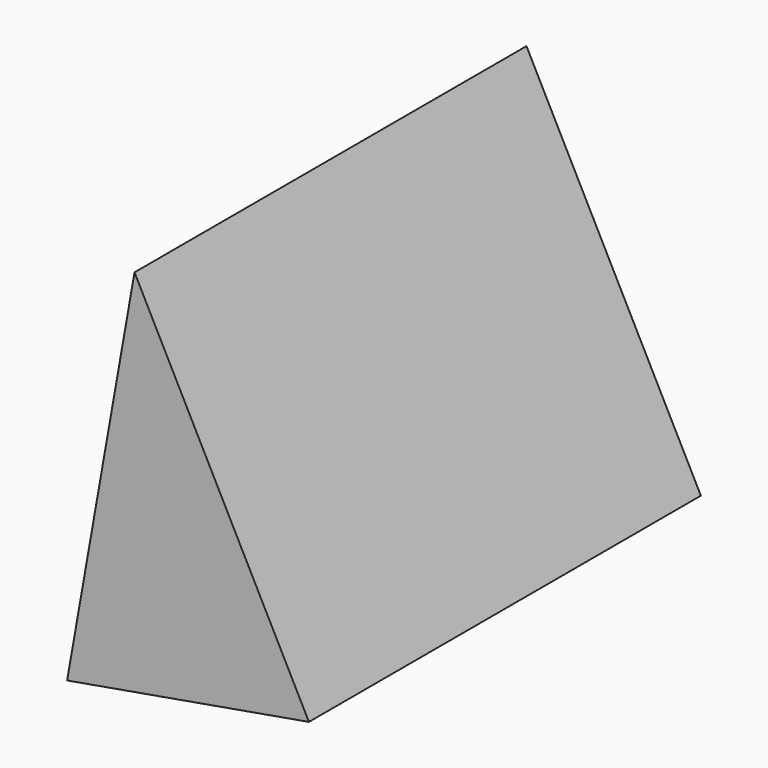
from build123d import *

# Parameters (mm, degrees)
F1_DEPTH = 77.216


# Not quite as in the source:
# - the program builds the solid bodies; features that only make, move or delete a surface that nothing else refers to are left out


with BuildPart() as f1:
    # F0 (on Front) → F1 (new body)
    with BuildSketch(Plane.XZ):
        Polygon((44.4227504639, -32.5769946799), (33.8973663747, 23.819770664), (23.2769409747, -36.2614902778), align=None)
        Polygon((61.3817200065, -29.6220239252), (33.8973663747, 23.819770664), (44.4227504639, -32.5769946799), align=None)
    extrude(amount=F1_DEPTH)


solid = f1.part
